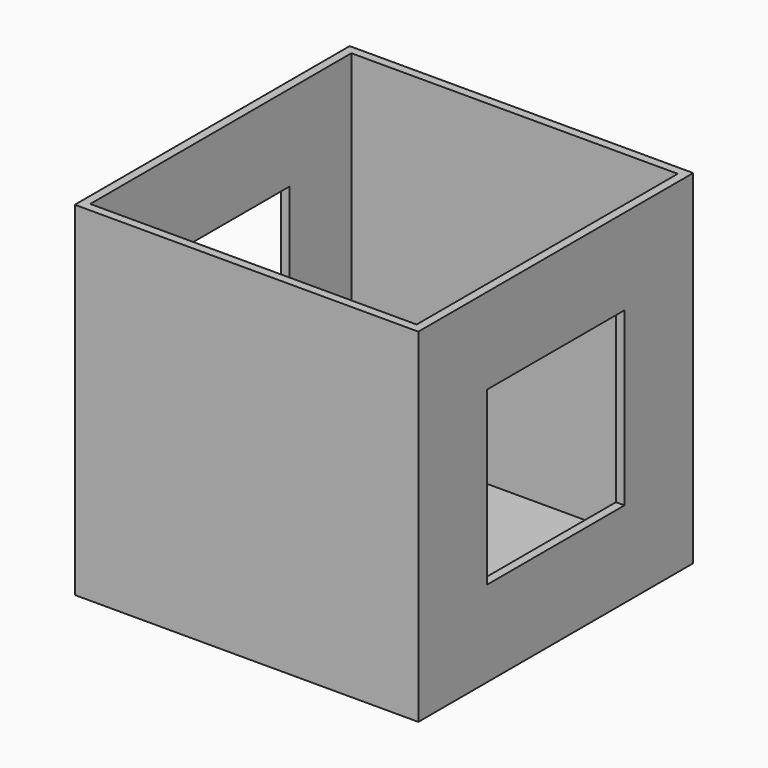
from build123d import *

# Parameters (mm, degrees)
F0_W     = 100
F0_H     = 100
F2_DEPTH = 50
F3_DEPTH = 50
F4_T     = -2.5
F8_DEPTH = 100.001


# Not quite as in the source:
# - a feature names something its author has since deleted; it is built from what else it names


with BuildPart() as f2:
    # F0 (on Front) → F2 (new body)
    with BuildSketch(Plane.XZ):
        with Locations((0, 50)):
            Rectangle(F0_W, F0_H)
    extrude(amount=F2_DEPTH)

    # F3 (add): a face of the model
    f3_faces = [f2.faces().sort_by_distance(p)[0] for p in [
        (0, 0, 50),
    ]]
    extrude(f3_faces, amount=F3_DEPTH)

    # F4
    f4_openings = [f2.faces().sort_by_distance(p)[0] for p in [
        (0, 0, 100),
    ]]
    offset(amount=F4_T, openings=f4_openings)

    # F7 (on offset) → F8 (cut, through all)
    with BuildSketch(Plane.YZ.offset(50)):
        Polygon((25, 75), (-25, 75), (-25, 25), (0, 25), (25, 25), align=None)
    extrude(amount=-F8_DEPTH, mode=Mode.SUBTRACT)


solid = f2.part
